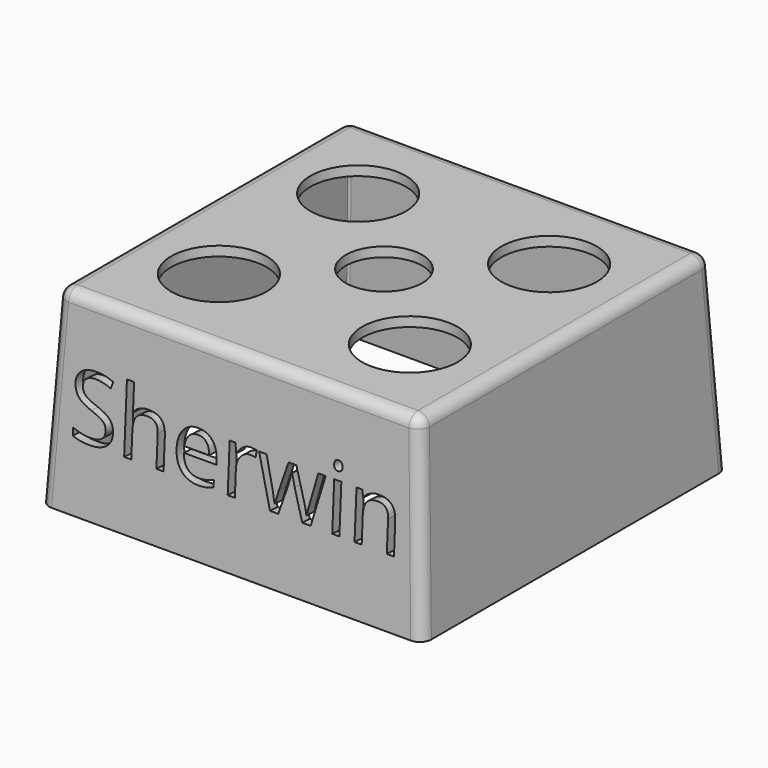
from build123d import *

# Parameters (mm, degrees)
F0_W         = 100
F0_H         = 100
F1_DEPTH     = 50
F1_TAPER     = 3
F2_R         = 3
F3_T         = -2.5
F4_R         = 10
F5_DEPTH     = 3
F4_R_2       = 12.5
F6_DEPTH     = 3
F7_TEXT_SIZE = 23.068071136
F8_DEPTH     = 3


# Not quite as in the source:
# - Text() gives the source's letters only with a copy of the font that has no kerning and outlines rounded to 1/6400 em; it was checked with that copy


with BuildPart() as f1:
    # F0 (on Top) → F1 (new body)
    with BuildSketch(Plane.XY):
        with Locations((50, 50)):
            Rectangle(F0_W, F0_H)
    extrude(amount=F1_DEPTH, taper=F1_TAPER)

    # F2
    f2_edges = [f1.edges().sort_by_distance(p)[0] for p in [
        (98.689806, 1.310194, 25),
        (2.620389, 50, 50),
        (50, 2.620389, 50),
        (97.379611, 50, 50),
        (50, 97.379611, 50),
        (98.689806, 98.689806, 25),
        (1.310194, 1.310194, 25),
        (1.310194, 98.689806, 25),
    ]]
    fillet(f2_edges, radius=F2_R)

    # F3
    f3_openings = [f1.faces().sort_by_distance(p)[0] for p in [
        (50, 50, 0),
    ]]
    offset(amount=F3_T, openings=f3_openings)

    # F4 (on face) → F5 (cut)
    with BuildSketch(Plane.XY.offset(50)):
        with Locations((50, 50)):
            Circle(F4_R)
    extrude(amount=-F5_DEPTH, mode=Mode.SUBTRACT)

    # F4 (on face) → F6 (cut)
    with BuildSketch(Plane.XY.offset(50)):
        with Locations((25.014026463, 27.2190853953)):
            Circle(F4_R_2)
        with Locations((74.985973537, 72.7809146047)):
            Circle(F4_R_2)
        with Locations((74.985973537, 27.2190853953)):
            Circle(F4_R_2)
        with Locations((25.014026463, 72.7809146047)):
            Circle(F4_R_2)
    extrude(amount=-F6_DEPTH, mode=Mode.SUBTRACT)

    # F7 (on face) → F8 (cut)
    with BuildSketch(Plane(origin=(0, 0, 0), x_dir=(1, 0, 0), z_dir=(0, -0.9986295348, 0.0523359562))):
        with Locations((6.6212131059, 17.3342693597)):
            Text('Sherwin', F7_TEXT_SIZE, font='Open Sans', text_align=(TextAlign.LEFT, TextAlign.BOTTOM))
    extrude(amount=-F8_DEPTH, mode=Mode.SUBTRACT)


solid = f1.part
